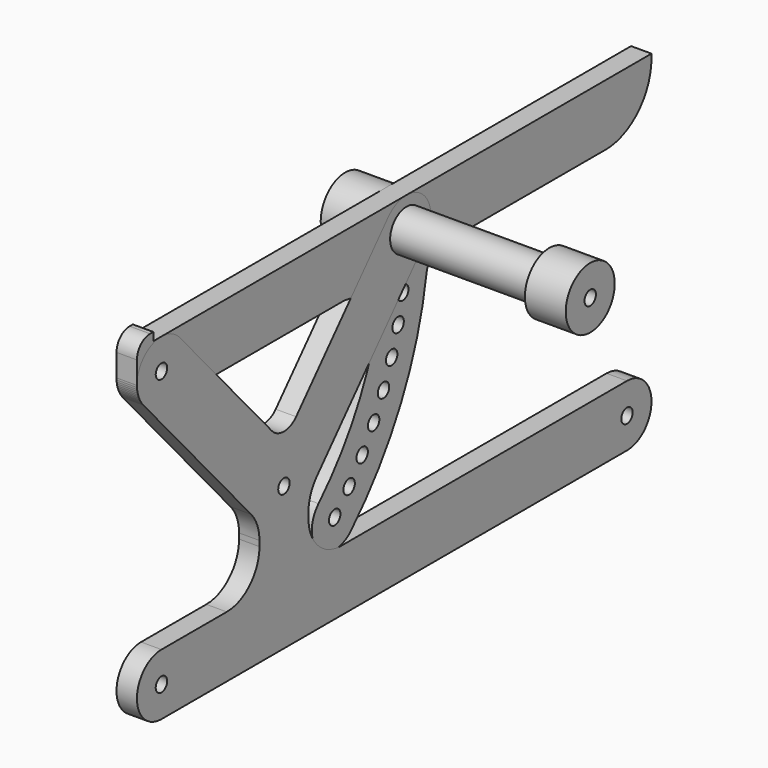
from build123d import *

# Parameters (mm, degrees)
F0_R      = 1.75
F1_DEPTH  = 5
F2_R      = 1.75
F3_DEPTH  = 5
F4_R      = 5
F5_DEPTH  = 40
F6_R      = 7.5
F7_DEPTH  = 10
F8_R      = 7.5
F9_DEPTH  = 10
F10_R     = 1.75
F11_DEPTH = 60.001


with BuildPart() as f1:
    # F0 (on Right) → F1 (new body)
    with BuildSketch(Plane.YZ):
        with BuildLine():
            Line((75, 7.5), (-75, 7.5))
            Line((-75, 7.5), (-77.5, 7.5))
            Line((-77.5, 7.5), (-77.5, 9.5))
            Line((-77.5, 9.5), (-78.5, 9.5))
            ThreePointArc((-78.5, 9.5), (-81.3284271247, 8.3284271247), (-82.5, 5.5))
            Line((-82.5, 5.5), (-82.5, 0))
            ThreePointArc((-82.5, 0), (-80.3033008589, -5.3033008589), (-75, -7.5))
            Line((-75, -7.5), (-19.7030742265, -7.5))
            ThreePointArc((-19.7030742265, -7.5), (-11.6354719249, -11.5912105213), (-10.1691215069, -20.5172413793))
            ThreePointArc((-10.1691215069, -20.5172413793), (-16.8848376732, -35.3076182675), (-26.9167388793, -48.0832611207))
            ThreePointArc((-26.9167388793, -48.0832611207), (-26.9167388793, -57.9827560573), (-17.0172439427, -57.9827560573))
            ThreePointArc((-17.0172439427, -57.9827560573), (-1.6988251739, -36.7551053475), (6.1492063101, -11.7816091954))
            ThreePointArc((6.1492063101, -11.7816091954), (7.8256283254, -8.7189978826), (11.0973286461, -7.5))
            Line((11.0973286461, -7.5), (61, -7.5))
            ThreePointArc((61, -7.5), (70.8994949366, -3.3994949366), (75, 6.5))
            Line((75, 6.5), (75, 7.5))
        make_face()
        with Locations((-21.966991411, -53.033008589)):
            Circle(F0_R, mode=Mode.SUBTRACT)
        with Locations((-17.5466667661, -48.2090707265)):
            Circle(F0_R, mode=Mode.SUBTRACT)
        with Locations((-13.5635966783, -43.0182327263)):
            Circle(F0_R, mode=Mode.SUBTRACT)
        with Locations((-10.0480947162, -37.5)):
            Circle(F0_R, mode=Mode.SUBTRACT)
        with Locations((-7.0269159723, -31.6963696306)):
            Circle(F0_R, mode=Mode.SUBTRACT)
        with Locations((-4.5230534411, -25.6515107494)):
            Circle(F0_R, mode=Mode.SUBTRACT)
        with Locations((-75, 0)):
            Circle(F0_R, mode=Mode.SUBTRACT)
        with Locations((-2.5555630283, -19.4114283827)):
            Circle(F0_R, mode=Mode.SUBTRACT)
        with Locations((-1.1394185241, -13.023613325)):
            Circle(F0_R, mode=Mode.SUBTRACT)
        Circle(F0_R, mode=Mode.SUBTRACT)
    extrude(amount=F1_DEPTH)


with BuildPart() as f3:
    # F2 (on Right) → F3 (new body)
    with BuildSketch(Plane.YZ):
        with BuildLine():
            Line((-41.2296883081, -26.5617544674), (-69.4054675378, 4.9951182698))
            ThreePointArc((-69.4054675378, 4.9951182698), (-79.9951182698, 5.5945324622), (-80.5945324622, -4.9951182698))
            Line((-80.5945324622, -4.9951182698), (-47.5406233837, -42.0154964377))
            ThreePointArc((-47.5406233837, -42.0154964377), (-45.6567198971, -45.1115109071), (-45, -48.6756541308))
            Line((-45, -48.6756541308), (-45, -50))
            ThreePointArc((-45, -50), (-47.9289321881, -57.0710678119), (-55, -60))
            Line((-55, -60), (-75, -60))
            ThreePointArc((-75, -60), (-82.5, -67.5), (-75, -75))
            Line((-75, -75), (67.5, -75))
            ThreePointArc((67.5, -75), (72.8033008589, -72.8033008589), (75, -67.5))
            ThreePointArc((75, -67.5), (72.8033008589, -62.1966991411), (67.5, -60))
            Line((67.5, -60), (-20, -60))
            ThreePointArc((-20, -60), (-27.0710678119, -57.0710678119), (-30, -50))
            Line((-30, -50), (-30, -48.6756541308))
            ThreePointArc((-30, -48.6756541308), (-29.3432801029, -45.1115109071), (-27.4593766163, -42.0154964377))
            Line((-27.4593766163, -42.0154964377), (5.5945324622, -4.9951182698))
            ThreePointArc((5.5945324622, -4.9951182698), (4.9951182698, 5.5945324622), (-5.5945324622, 4.9951182698))
            Line((-5.5945324622, 4.9951182698), (-33.7703116919, -26.5617544674))
            ThreePointArc((-33.7703116919, -26.5617544674), (-37.5, -28.2316756209), (-41.2296883081, -26.5617544674))
        make_face()
        with Locations((-75, -67.5)):
            Circle(F2_R, mode=Mode.SUBTRACT)
        with Locations((-37.5, -40)):
            Circle(F2_R, mode=Mode.SUBTRACT)
        with Locations((67.5, -67.5)):
            Circle(F2_R, mode=Mode.SUBTRACT)
        with Locations((-75, 0)):
            Circle(F2_R, mode=Mode.SUBTRACT)
        Circle(F2_R, mode=Mode.SUBTRACT)
    extrude(amount=F3_DEPTH)


with BuildPart() as f5:
    # F4 (on Right) → F5 (new body)
    with BuildSketch(Plane.YZ):
        Circle(F4_R)
    extrude(amount=F5_DEPTH)

    # F6 (on face) → F7 (join)
    with BuildSketch(Plane.YZ.offset(40)):
        Circle(F6_R)
    extrude(amount=F7_DEPTH)

    # F8 (on face) → F9 (join)
    with BuildSketch(Plane(origin=(0, 0, 0), x_dir=(0, -1, 0), z_dir=(-1, 0, 0))):
        Circle(F8_R)
    extrude(amount=F9_DEPTH)

    # F10 (on face) → F11 (cut, through all)
    with BuildSketch(Plane(origin=(-10, 0, 0), x_dir=(0, -1, 0), z_dir=(-1, 0, 0))):
        Circle(F10_R)
    extrude(amount=-F11_DEPTH, mode=Mode.SUBTRACT)


solid = Compound([f1.part, f3.part, f5.part])
